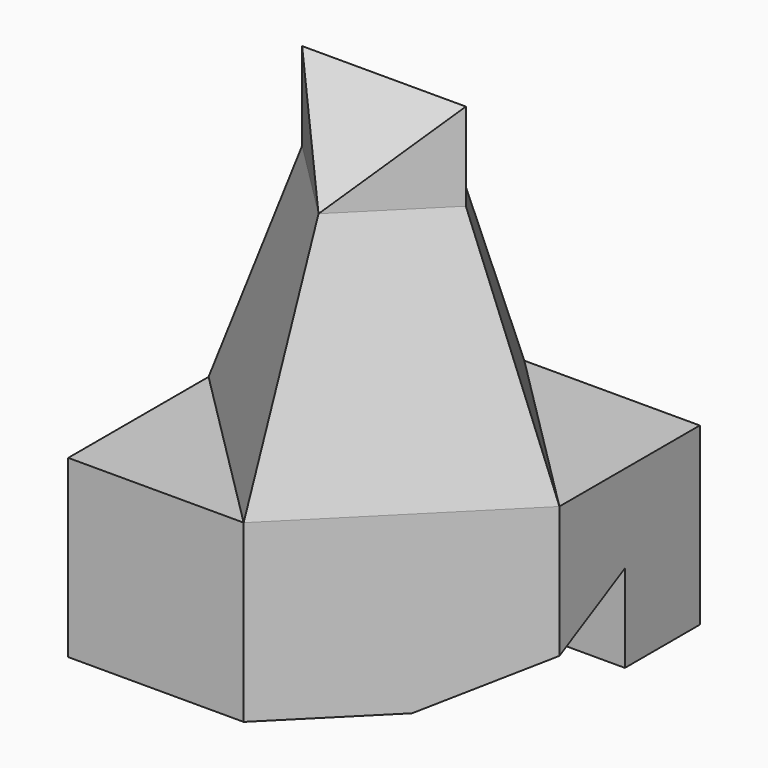
from build123d import *

# Parameters (mm, degrees)
F0_W          = 60
F0_H          = 60
F1_DEPTH      = 30
F6_DEPTH      = 15
F8_DEPTH      = 14.001
F8_DEPTH_BACK = 14.001
F9_DEPTH      = 30.001
F19_DEPTH     = 60


with BuildPart() as f1:
    # F0 (on Top) → F1 (new body)
    with BuildSketch(Plane.XY):
        Rectangle(F0_W, F0_H)
    extrude(amount=F1_DEPTH)

    # F2 (on face) → F5 section 0
    with BuildSketch(Plane.XY.offset(30)):
        Polygon((30, 0), (0, 30), (-30, 0), (0, -30), align=None)
    # F4 (on offset) → F5 section 1
    with BuildSketch(Plane.XY.offset(70)):
        Polygon((14, 0), (0, 14), (-14, 0), (0, -14), align=None)
    loft()

    # F6 (add): a face of the model
    f6_faces = [f1.faces().sort_by_distance(p)[0] for p in [
        (0, 0, 70),
    ]]
    extrude(f6_faces, amount=F6_DEPTH)

    # F7 (on Right) → F8 (cut, two sides)
    with BuildSketch(Plane.YZ) as f8_sk:
        Polygon((14, 85), (0, 85), (14, 70), align=None)
        Polygon((0, 85), (-14, 85), (-14, 70), align=None)
    extrude(amount=-F8_DEPTH, mode=Mode.SUBTRACT)
    extrude(f8_sk.sketch, amount=F8_DEPTH_BACK, mode=Mode.SUBTRACT)

    # F9 (cut, through all): a face of the model
    f9_faces = [f1.faces().sort_by_distance(p)[0] for p in [
        (20, -20, 30),
    ]]
    extrude(f9_faces, amount=-F9_DEPTH, mode=Mode.SUBTRACT)

    # F13 (on offset) → F17 section 0
    with BuildSketch(Plane.YZ.offset(-14)):
        Polygon((14, -5), (14, 0), (14, 30), (-14, 15), (-14, 0), (-14, -5), align=None)
    # F11 (on offset) → F17 section 1
    with BuildSketch(Plane.YZ.offset(14)):
        Polygon((14, 15), (-14, 0), (-14, -5), (14, -5), (14, 0), align=None)
    loft(mode=Mode.SUBTRACT)

    # F18 (on face) → F19 (cut, through all)
    with BuildSketch(Plane.YZ.offset(30)):
        Polygon((14, 0), (14, 15), (0, 7.5), (0, 0), align=None)
        Polygon((0, 0), (0, 7.5), (-14, 0), align=None)
    extrude(amount=-F19_DEPTH, mode=Mode.SUBTRACT)


solid = f1.part
